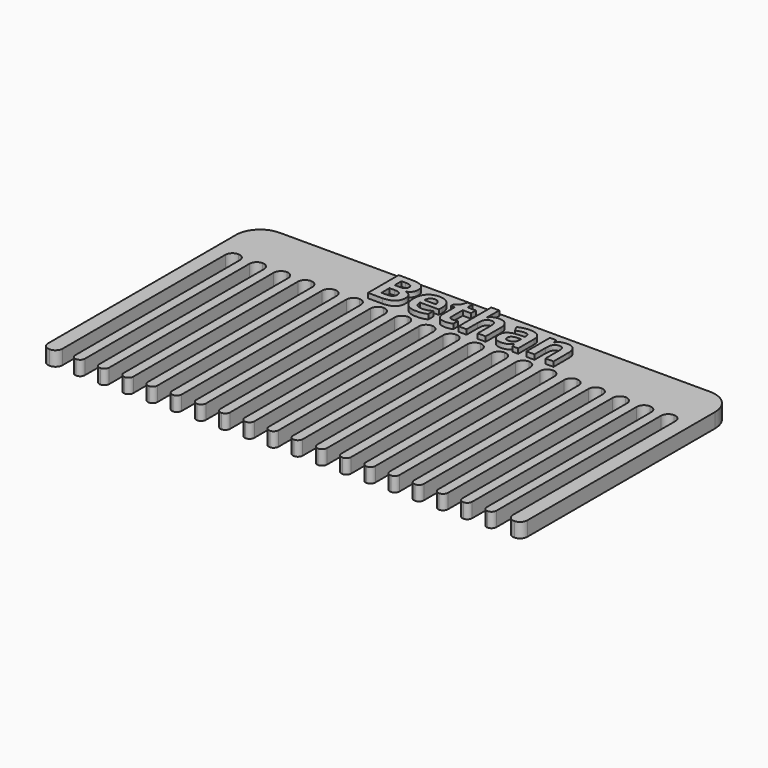
from build123d import *

# Parameters (mm, degrees)
F1_DEPTH     = 3
F2_TEXT_SIZE = 11.1111111111
F3_DEPTH     = 1


# Not quite as in the source:
# - Text() gives the source's letters only with a copy of the font that has no kerning and outlines rounded to 1/6400 em; it was checked with that copy


with BuildPart() as f1:
    # F0 (on Top) → F1 (new body)
    with BuildSketch(Plane.XY):
        with BuildLine():
            Line((0, 50), (0, 1.5))
            ThreePointArc((0, 1.5), (0.4393398282, 0.4393398282), (1.5, 0))
            ThreePointArc((1.5, 0), (2.5606601718, 0.4393398282), (3, 1.5))
            Line((3, 1.5), (3, 43.5))
            ThreePointArc((3, 43.5), (3.4393398282, 44.5606601718), (4.5, 45))
            ThreePointArc((4.5, 45), (5.5606601718, 44.5606601718), (6, 43.5))
            Line((6, 43.5), (6, 1))
            ThreePointArc((6, 1), (6.2928932188, 0.2928932188), (7, 0))
            ThreePointArc((7, 0), (7.7071067812, 0.2928932188), (8, 1))
            Line((8, 1), (8, 43.5))
            ThreePointArc((8, 43.5), (8.4393398282, 44.5606601718), (9.5, 45))
            ThreePointArc((9.5, 45), (10.5606601718, 44.5606601718), (11, 43.5))
            Line((11, 43.5), (11, 1))
            ThreePointArc((11, 1), (11.2928932188, 0.2928932188), (12, 0))
            ThreePointArc((12, 0), (12.7071067812, 0.2928932188), (13, 1))
            Line((13, 1), (13, 43.5))
            ThreePointArc((13, 43.5), (13.4393398282, 44.5606601718), (14.5, 45))
            ThreePointArc((14.5, 45), (15.5606601718, 44.5606601718), (16, 43.5))
            Line((16, 43.5), (16, 1))
            ThreePointArc((16, 1), (16.2928932188, 0.2928932188), (17, 0))
            ThreePointArc((17, 0), (17.7071067812, 0.2928932188), (18, 1))
            Line((18, 1), (18, 43.5))
            ThreePointArc((18, 43.5), (18.4393398282, 44.5606601718), (19.5, 45))
            ThreePointArc((19.5, 45), (20.5606601718, 44.5606601718), (21, 43.5))
            Line((21, 43.5), (21, 1))
            ThreePointArc((21, 1), (21.2928932188, 0.2928932188), (22, 0))
            ThreePointArc((22, 0), (22.7071067812, 0.2928932188), (23, 1))
            Line((23, 1), (23, 43.5))
            ThreePointArc((23, 43.5), (23.4393398282, 44.5606601718), (24.5, 45))
            ThreePointArc((24.5, 45), (25.5606601718, 44.5606601718), (26, 43.5))
            Line((26, 43.5), (26, 1))
            ThreePointArc((26, 1), (26.2928932188, 0.2928932188), (27, 0))
            ThreePointArc((27, 0), (27.7071067812, 0.2928932188), (28, 1))
            Line((28, 1), (28, 43.5))
            ThreePointArc((28, 43.5), (28.4393398282, 44.5606601718), (29.5, 45))
            ThreePointArc((29.5, 45), (30.5606601718, 44.5606601718), (31, 43.5))
            Line((31, 43.5), (31, 1))
            ThreePointArc((31, 1), (31.2928932188, 0.2928932188), (32, 0))
            ThreePointArc((32, 0), (32.7071067812, 0.2928932188), (33, 1))
            Line((33, 1), (33, 43.5))
            ThreePointArc((33, 43.5), (33.4393398282, 44.5606601718), (34.5, 45))
            ThreePointArc((34.5, 45), (35.5606601718, 44.5606601718), (36, 43.5))
            Line((36, 43.5), (36, 1))
            ThreePointArc((36, 1), (36.2928932188, 0.2928932188), (37, 0))
            ThreePointArc((37, 0), (37.7071067812, 0.2928932188), (38, 1))
            Line((38, 1), (38, 43.5))
            ThreePointArc((38, 43.5), (38.4393398282, 44.5606601718), (39.5, 45))
            ThreePointArc((39.5, 45), (40.5606601718, 44.5606601718), (41, 43.5))
            Line((41, 43.5), (41, 1))
            ThreePointArc((41, 1), (41.2928932188, 0.2928932188), (42, 0))
            ThreePointArc((42, 0), (42.7071067812, 0.2928932188), (43, 1))
            Line((43, 1), (43, 43.5))
            ThreePointArc((43, 43.5), (43.4393398282, 44.5606601718), (44.5, 45))
            ThreePointArc((44.5, 45), (45.5606601718, 44.5606601718), (46, 43.5))
            Line((46, 43.5), (46, 1))
            ThreePointArc((46, 1), (46.2928932188, 0.2928932188), (47, 0))
            ThreePointArc((47, 0), (47.7071067812, 0.2928932188), (48, 1))
            Line((48, 1), (48, 43.5))
            ThreePointArc((48, 43.5), (48.4393398282, 44.5606601718), (49.5, 45))
            ThreePointArc((49.5, 45), (50.5606601718, 44.5606601718), (51, 43.5))
            Line((51, 43.5), (51, 1))
            ThreePointArc((51, 1), (51.2928932188, 0.2928932188), (52, 0))
            ThreePointArc((52, 0), (52.7071067812, 0.2928932188), (53, 1))
            Line((53, 1), (53, 43.5))
            ThreePointArc((53, 43.5), (53.4393398282, 44.5606601718), (54.5, 45))
            ThreePointArc((54.5, 45), (55.5606601718, 44.5606601718), (56, 43.5))
            Line((56, 43.5), (56, 1))
            ThreePointArc((56, 1), (56.2928932188, 0.2928932188), (57, 0))
            ThreePointArc((57, 0), (57.7071067812, 0.2928932188), (58, 1))
            Line((58, 1), (58, 43.5))
            ThreePointArc((58, 43.5), (58.4393398282, 44.5606601718), (59.5, 45))
            ThreePointArc((59.5, 45), (60.5606601718, 44.5606601718), (61, 43.5))
            Line((61, 43.5), (61, 1))
            ThreePointArc((61, 1), (61.2928932188, 0.2928932188), (62, 0))
            ThreePointArc((62, 0), (62.7071067812, 0.2928932188), (63, 1))
            Line((63, 1), (63, 43.5))
            ThreePointArc((63, 43.5), (63.4393398282, 44.5606601718), (64.5, 45))
            ThreePointArc((64.5, 45), (65.5606601718, 44.5606601718), (66, 43.5))
            Line((66, 43.5), (66, 1))
            ThreePointArc((66, 1), (66.2928932188, 0.2928932188), (67, 0))
            ThreePointArc((67, 0), (67.7071067812, 0.2928932188), (68, 1))
            Line((68, 1), (68, 43.5))
            ThreePointArc((68, 43.5), (68.4393398282, 44.5606601718), (69.5, 45))
            ThreePointArc((69.5, 45), (70.5606601718, 44.5606601718), (71, 43.5))
            Line((71, 43.5), (71, 1))
            ThreePointArc((71, 1), (71.2928932188, 0.2928932188), (72, 0))
            ThreePointArc((72, 0), (72.7071067812, 0.2928932188), (73, 1))
            Line((73, 1), (73, 43.5))
            ThreePointArc((73, 43.5), (73.4393398282, 44.5606601718), (74.5, 45))
            ThreePointArc((74.5, 45), (75.5606601718, 44.5606601718), (76, 43.5))
            Line((76, 43.5), (76, 1))
            ThreePointArc((76, 1), (76.2928932188, 0.2928932188), (77, 0))
            ThreePointArc((77, 0), (77.7071067812, 0.2928932188), (78, 1))
            Line((78, 1), (78, 43.5))
            ThreePointArc((78, 43.5), (78.4393398282, 44.5606601718), (79.5, 45))
            ThreePointArc((79.5, 45), (80.5606601718, 44.5606601718), (81, 43.5))
            Line((81, 43.5), (81, 1))
            ThreePointArc((81, 1), (81.2928932188, 0.2928932188), (82, 0))
            ThreePointArc((82, 0), (82.7071067812, 0.2928932188), (83, 1))
            Line((83, 1), (83, 43.5))
            ThreePointArc((83, 43.5), (83.4393398282, 44.5606601718), (84.5, 45))
            ThreePointArc((84.5, 45), (85.5606601718, 44.5606601718), (86, 43.5))
            Line((86, 43.5), (86, 1))
            ThreePointArc((86, 1), (86.2928932188, 0.2928932188), (87, 0))
            ThreePointArc((87, 0), (87.7071067812, 0.2928932188), (88, 1))
            Line((88, 1), (88, 43.5))
            ThreePointArc((88, 43.5), (88.4393398282, 44.5606601718), (89.5, 45))
            ThreePointArc((89.5, 45), (90.5606601718, 44.5606601718), (91, 43.5))
            Line((91, 43.5), (91, 1))
            ThreePointArc((91, 1), (91.2928932188, 0.2928932188), (92, 0))
            ThreePointArc((92, 0), (92.7071067812, 0.2928932188), (93, 1))
            Line((93, 1), (93, 43.5))
            ThreePointArc((93, 43.5), (93.4393398282, 44.5606601718), (94.5, 45))
            ThreePointArc((94.5, 45), (95.5606601718, 44.5606601718), (96, 43.5))
            Line((96, 43.5), (96, 1.5))
            ThreePointArc((96, 1.5), (96.4393398282, 0.4393398282), (97.5, 0))
            ThreePointArc((97.5, 0), (98.5606601718, 0.4393398282), (99, 1.5))
            Line((99, 1.5), (99, 50))
            ThreePointArc((99, 50), (97.5355339059, 53.5355339059), (94, 55))
            Line((94, 55), (49.5, 55))
            Line((49.5, 55), (5, 55))
            ThreePointArc((5, 55), (1.4644660941, 53.5355339059), (0, 50))
        make_face()
    extrude(amount=F1_DEPTH)

    # F2 (on face) → F3 (join)
    with BuildSketch(Plane.XY.offset(3)):
        with Locations((29.4730902778, 46)):
            Text('Bethan', F2_TEXT_SIZE, font='Open Sans', font_style=FontStyle.BOLD, text_align=(TextAlign.LEFT, TextAlign.BOTTOM))
    extrude(amount=F3_DEPTH)


solid = f1.part
